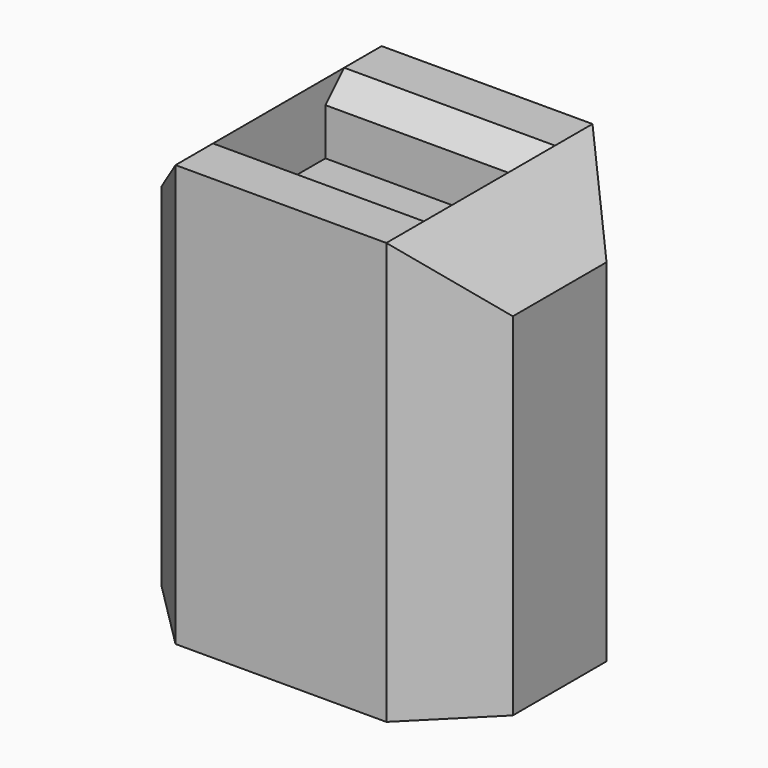
from build123d import *

# Parameters (mm, degrees)
F0_W     = 45
F0_H     = 25
F1_DEPTH = 75
F2_DEPTH = 90
F3_SIZE  = 14.99999
F4_SIZE  = 5


# Not quite as in the source:
# - a fillet or chamfer is up to 0.001 mm smaller than in the source, because OpenCascade refuses the exact size


with BuildPart() as f1:
    # F0 (on Top) → F1 (new body)
    with BuildSketch(Plane.XY):
        Rectangle(F0_W, F0_H)
    extrude(amount=F1_DEPTH)

    # F0 (on Top) → F2 (join)
    with BuildSketch(Plane.XY):
        Polygon((37.5, 27.5), (-37.5, 27.5), (-37.5, -27.5), (-22.5, -27.5), (22.5, -27.5), (37.5, -27.5), align=None)
        Rectangle(F0_W, F0_H, mode=Mode.SUBTRACT)
    extrude(amount=F2_DEPTH)

    # F3 (size 15 in the source; OpenCascade refuses exactly that, so slightly less here)
    f3_edges = [f1.edges().sort_by_distance(p)[0] for p in [
        (-37.5, 0, 90),
        (37.5, 0, 90),
        (37.5, 27.5, 45),
        (37.5, -27.5, 45),
        (-37.5, -27.5, 45),
        (-37.5, 27.5, 45),
    ]]
    chamfer(f3_edges, length=F3_SIZE)

    # F4
    f4_edges = [f1.edges().sort_by_distance(p)[0] for p in [
        (0, 12.5, 90),
        (0, -12.5, 90),
    ]]
    chamfer(f4_edges, length=F4_SIZE)


solid = f1.part
